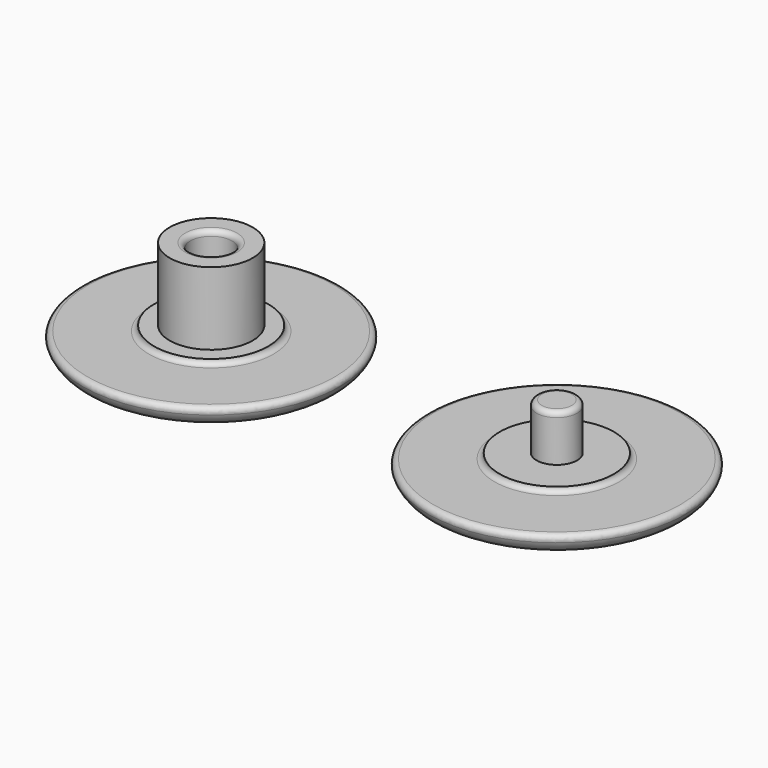
from build123d import *

# Parameters (mm, degrees)
F0_R     = 12.5
F0_R_2   = 5.5
F1_DEPTH = 2
F0_R_3   = 4
F2_DEPTH = 2.5
F0_R_4   = 1.95
F0_R_5   = 2
F3_DEPTH = 9.5
F4_DEPTH = 7
F7_R     = 1.99999
F8_R     = 0.49999


# Not quite as in the source:
# - a fillet or chamfer is up to 0.001 mm smaller than in the source, because OpenCascade refuses the exact size


with BuildPart() as f1:
    # F0 (on Top) → F1 (new body)
    with BuildSketch(Plane.XY):
        with Locations((-165.7585352659, 137.4950408936)):
            Circle(F0_R)
        with Locations((-165.7585352659, 137.4950408936)):
            Circle(F0_R_2, mode=Mode.SUBTRACT)
    extrude(amount=F1_DEPTH)


with BuildPart() as f1b:
    # F0 (on Top) → F1, piece 2 (new body)
    with BuildSketch(Plane.XY):
        with Locations((-132.4781477451, 137.4950408936)):
            Circle(F0_R)
        with Locations((-132.4781477451, 137.4950408936)):
            Circle(F0_R_2, mode=Mode.SUBTRACT)
    extrude(amount=F1_DEPTH)


with BuildPart() as f2:
    # F0 (on Top) → F2 (new body)
    with BuildSketch(Plane.XY):
        with Locations((-165.7585352659, 137.4950408936)):
            Circle(F0_R_2)
        with Locations((-165.7585352659, 137.4950408936)):
            Circle(F0_R_3, mode=Mode.SUBTRACT)
    extrude(amount=F2_DEPTH)


with BuildPart() as f2b:
    # F0 (on Top) → F2, piece 2 (new body)
    with BuildSketch(Plane.XY):
        with Locations((-132.4781477451, 137.4950408936)):
            Circle(F0_R_2)
        with Locations((-132.4781477451, 137.4950408936)):
            Circle(F0_R_4, mode=Mode.SUBTRACT)
    extrude(amount=F2_DEPTH)

    # F0 (on Top) → F4 (join)
    with BuildSketch(Plane.XY):
        with Locations((-132.4781477451, 137.4950408936)):
            Circle(F0_R_4)
    extrude(amount=F4_DEPTH)


with BuildPart() as f2c:
    # F0 (on Top) → F2, piece 3 (new body)
    with BuildSketch(Plane.XY):
        with Locations((-165.7585352659, 137.4950408936)):
            Circle(F0_R_5)
    extrude(amount=F2_DEPTH)


with BuildPart() as f3:
    # F0 (on Top) → F3 (new body)
    with BuildSketch(Plane.XY):
        with Locations((-165.7585352659, 137.4950408936)):
            Circle(F0_R_3)
        with Locations((-165.7585352659, 137.4950408936)):
            Circle(F0_R_5, mode=Mode.SUBTRACT)
    extrude(amount=F3_DEPTH)

    # F5: union F2c, F1, F2
    add(f2c.part)
    add(f1.part)
    add(f2.part)

    # F6: union F2b, F1b
    add(f2b.part)
    add(f1b.part)

    # F7 (radius 2 in the source; OpenCascade refuses exactly that, so slightly less here)
    f7_edges = [f3.edges().sort_by_distance(p)[0] for p in [
        (-144.978148, 137.495041, 0),
        (-178.258535, 137.495041, 0),
    ]]
    fillet(f7_edges, radius=F7_R)

    # F8 (radius 0.5 in the source; OpenCascade refuses exactly that, so slightly less here)
    f8_edges = [f3.edges().sort_by_distance(p)[0] for p in [
        (-178.258535, 137.495041, 2),
        (-171.258535, 137.495041, 2),
        (-144.978148, 137.495041, 2),
        (-137.978148, 137.495041, 2),
        (-134.428148, 137.495041, 7),
        (-167.758535, 137.495041, 9.5),
    ]]
    fillet(f8_edges, radius=F8_R)


solid = f3.part
